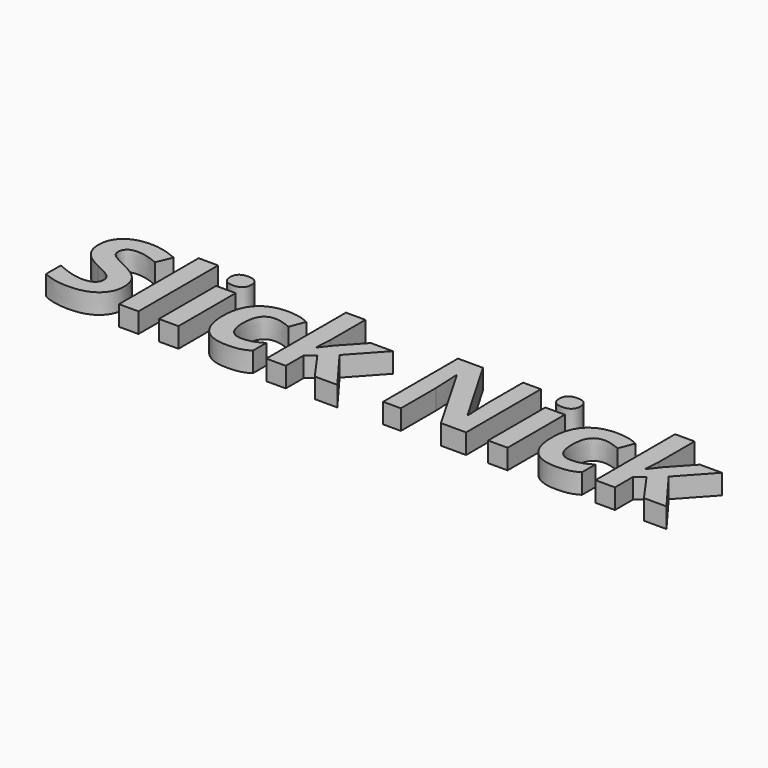
from build123d import *

# Parameters (mm, degrees)
F0_TEXT_SIZE = 20.8510501844
F1_DEPTH     = 3.175


# Not quite as in the source:
# - Text() gives the source's letters only with a copy of the font that has no kerning and outlines rounded to 1/6400 em; it was checked with that copy


with BuildPart() as f1:
    # F0 (on Top) → F1 (new body)
    with BuildSketch(Plane.XY):
        with Locations((-50.8, -6.8608144383)):
            Text('Slick Nick', F0_TEXT_SIZE, font='Open Sans', font_style=FontStyle.BOLD, text_align=(TextAlign.LEFT, TextAlign.BOTTOM))
    extrude(amount=F1_DEPTH)


solid = f1.part
